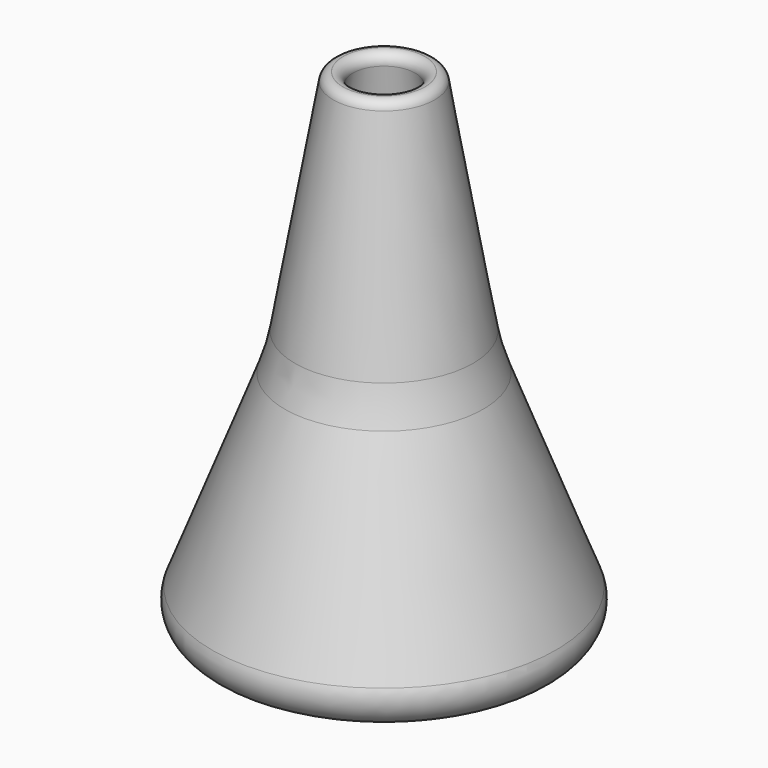
from build123d import *

# Parameters (mm, degrees)
F3_R = 1.5
F2_R = 5
F5_R = 1.5
F6_R = 0.5
F7_R = 10


with BuildPart() as f1:
    # F0 (on Right) → F1 (revolve)
    with BuildSketch(Plane.YZ):
        Polygon((-9.5, 0), (0, 0), (0, 25), (-2.5, 25), (-4.683943931, 12.5), align=None)
    revolve(axis=Axis((0, 0, 12.5), (0, 0, 1)))

    # F3 (on face) → F4 section 0
    with BuildSketch(Plane.XY.offset(25)):
        Circle(F3_R)
    # F2 (on face) → F4 section 1
    with BuildSketch(Plane(origin=(0, 0, 0), x_dir=(1, 0, 0), z_dir=(0, 0, -1))):
        Circle(F2_R)
    loft(mode=Mode.SUBTRACT)

    # F5
    f5_edges = [f1.edges().sort_by_distance(p)[0] for p in [
        (0, 9.5, 0),
    ]]
    fillet(f5_edges, radius=F5_R)

    # F6
    f6_edges = [f1.edges().sort_by_distance(p)[0] for p in [
        (-5, 0, 0),
        (0, 2.5, 25),
        (-1.5, 0, 25),
    ]]
    fillet(f6_edges, radius=F6_R)

    # F7
    f7_edges = [f1.edges().sort_by_distance(p)[0] for p in [
        (0, 4.683944, 12.5),
    ]]
    fillet(f7_edges, radius=F7_R)


solid = f1.part
